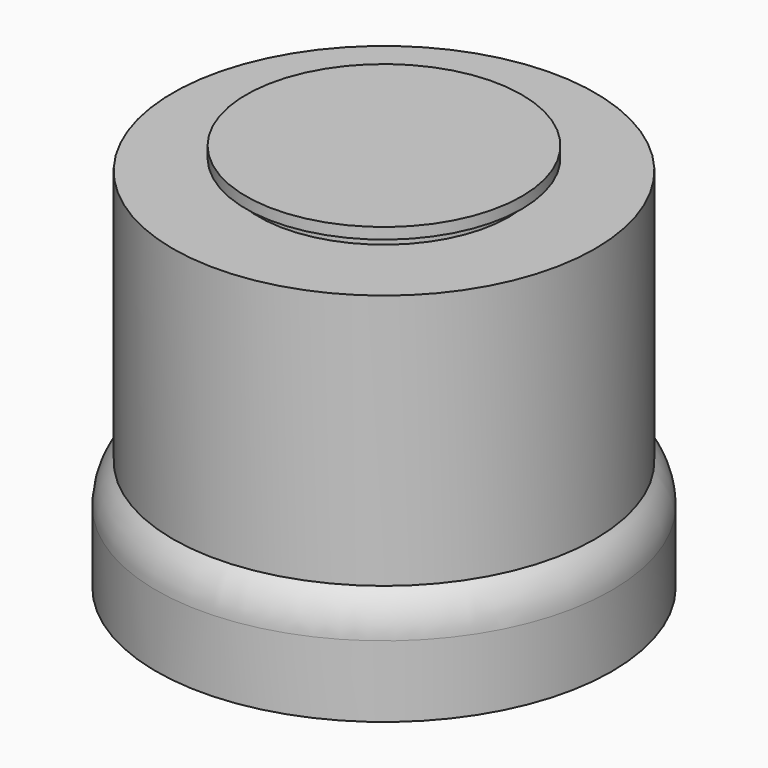
from build123d import *

# Parameters (mm, degrees)
F0_R     = 5.207
F1_DEPTH = 2.54
F2_R     = 4.826
F3_DEPTH = 5.842
F5_R     = 2.8575
F6_DEPTH = 0.254
F7_R     = 3.1496
F8_DEPTH = 0.254


# Not quite as in the source:
# - a fillet or chamfer that OpenCascade refuses, or shapes differently, is made with other operations: its cross-section is extruded or revolved along the edge and cut away or added


with BuildPart() as f1:
    # F0 (on Top) → F1 (new body)
    with BuildSketch(Plane.XY):
        Circle(F0_R)
    extrude(amount=F1_DEPTH)

    # F2 (on face) → F3 (join)
    with BuildSketch(Plane.XY.offset(2.54)):
        Circle(F2_R)
    extrude(amount=F3_DEPTH)

    # F4: fillet of radius 1.27 on 1 edges, made by hand

    # F4_s1 → F4_t2 (revolve, cut)
    with BuildSketch(Plane.XZ):
        with BuildLine():
            ThreePointArc((5.207, 1.6330385896), (5.1078821461, 2.1249074745), (4.826, 2.54))
            Line((4.826, 2.54), (5.207, 2.54))
            Line((5.207, 2.54), (5.207, 1.6330385896))
        make_face()
    revolve(axis=Axis((0, 0, 2.54), (0, 0, 1)), mode=Mode.SUBTRACT)

    # F5 (on face) → F6 (join)
    with BuildSketch(Plane.XY.offset(8.382)):
        Circle(F5_R)
    extrude(amount=F6_DEPTH)

    # F7 (on face) → F8 (join)
    with BuildSketch(Plane.XY.offset(8.636)):
        Circle(F7_R)
    extrude(amount=F8_DEPTH)


solid = f1.part
